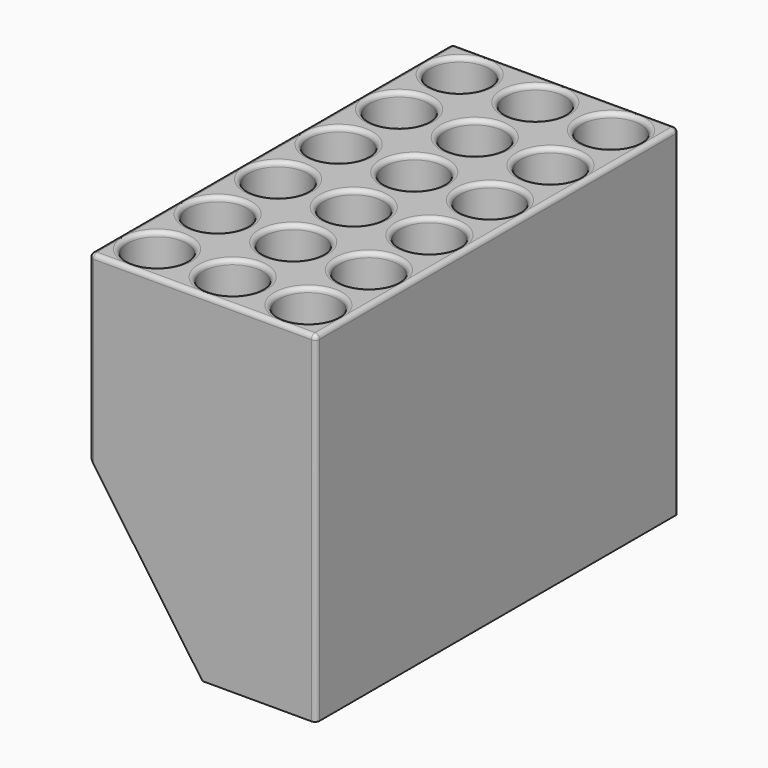
from build123d import *

# Parameters (mm, degrees)
F1_DEPTH     = 100
F2_R         = 6.5
F3_DEPTH     = 60
F4_R         = 6.5
F5_DEPTH     = 60
F6_R         = 6.5
F7_DEPTH     = 37
F8_T1_DEPTH  = 98
F8_T3_DEPTH  = 48
F8_T5_DEPTH  = 76.5
F8_T7_DEPTH  = 40.7962998314
F8_S11_W     = 1
F8_S11_H     = 1
F8_T12_DEPTH = 1
F8_S17_W     = 1
F8_S17_H     = 1
F8_T18_DEPTH = 1
F8_S23_W     = 1
F8_S23_H     = 1
F8_T24_DEPTH = 1
F8_S29_W     = 1
F8_S29_H     = 1
F8_T30_DEPTH = 1


# Not quite as in the source:
# - a fillet or chamfer that OpenCascade refuses, or shapes differently, is made with other operations: its cross-section is extruded or revolved along the edge and cut away or added


with BuildPart() as f1:
    # F0 (on Front) → F1 (new body)
    with BuildSketch(Plane.XZ):
        Polygon((0, 35.7037001686), (25, 0), (50, 0), (50, 75), (0, 75), align=None)
    extrude(amount=F1_DEPTH)

    # F2 (on face) → F3 (cut)
    with BuildSketch(Plane.XY.offset(75)):
        with Locations((41.667, -8.333)):
            Circle(F2_R)
        with Locations((41.667, -25)):
            Circle(F2_R)
        with Locations((41.667, -41.667)):
            Circle(F2_R)
        with Locations((41.667, -58.334)):
            Circle(F2_R)
        with Locations((41.667, -75.001)):
            Circle(F2_R)
        with Locations((41.667, -91.668)):
            Circle(F2_R)
    extrude(amount=-F3_DEPTH, mode=Mode.SUBTRACT)

    # F4 (on face) → F5 (cut)
    with BuildSketch(Plane.XY.offset(75)):
        with Locations((25, -8.333)):
            Circle(F4_R)
        with Locations((25, -25)):
            Circle(F4_R)
        with Locations((25, -41.667)):
            Circle(F4_R)
        with Locations((25, -58.334)):
            Circle(F4_R)
        with Locations((25, -75.001)):
            Circle(F4_R)
        with Locations((25, -91.668)):
            Circle(F4_R)
    extrude(amount=-F5_DEPTH, mode=Mode.SUBTRACT)

    # F6 (on face) → F7 (cut)
    with BuildSketch(Plane.XY.offset(75)):
        with Locations((8.333, -8.333)):
            Circle(F6_R)
        with Locations((8.333, -25)):
            Circle(F6_R)
        with Locations((8.333, -41.667)):
            Circle(F6_R)
        with Locations((8.333, -58.334)):
            Circle(F6_R)
        with Locations((8.333, -75.001)):
            Circle(F6_R)
        with Locations((8.333, -91.668)):
            Circle(F6_R)
    extrude(amount=-F7_DEPTH, mode=Mode.SUBTRACT)

    # F8: fillet of radius 1 on 26 edges, made by hand

    # F8_s2 → F8_t1 (cut)
    with BuildSketch(Plane.XZ.offset(1)):
        with BuildLine():
            ThreePointArc((49, 75), (49.7071067812, 74.7071067812), (50, 74))
            Line((50, 74), (50, 75))
            Line((50, 75), (49, 75))
        make_face()
        with BuildLine():
            ThreePointArc((0, 74), (0.2928932188, 74.7071067812), (1, 75))
            Line((1, 75), (0, 75))
            Line((0, 75), (0, 74))
        make_face()
    extrude(amount=F8_T1_DEPTH, mode=Mode.SUBTRACT)

    # F8_s4 → F8_t3 (cut)
    with BuildSketch(Plane.YZ.offset(1)):
        with BuildLine():
            ThreePointArc((0, 74), (-0.2928932188, 74.7071067812), (-1, 75))
            Line((-1, 75), (0, 75))
            Line((0, 75), (0, 74))
        make_face()
        with BuildLine():
            ThreePointArc((-100, 74), (-99.7071067812, 74.7071067812), (-99, 75))
            Line((-99, 75), (-100, 75))
            Line((-100, 75), (-100, 74))
        make_face()
    extrude(amount=F8_T3_DEPTH, mode=Mode.SUBTRACT)

    # F8_s6 → F8_t5 (cut)
    with BuildSketch(Plane.XY.offset(-2.5)):
        with BuildLine():
            ThreePointArc((49, -100), (49.7071067812, -99.7071067812), (50, -99))
            Line((50, -99), (50, -100))
            Line((50, -100), (49, -100))
        make_face()
        with BuildLine():
            ThreePointArc((49, 0), (49.7071067812, -0.2928932188), (50, -1))
            Line((50, -1), (50, 0))
            Line((50, 0), (49, 0))
        make_face()
    extrude(amount=F8_T5_DEPTH, mode=Mode.SUBTRACT)

    # F8_s8 → F8_t7 (cut)
    with BuildSketch(Plane.XY.offset(33.2037001686)):
        with BuildLine():
            ThreePointArc((0, -99), (0.2928932188, -99.7071067812), (1, -100))
            Line((1, -100), (0, -100))
            Line((0, -100), (0, -99))
        make_face()
        with BuildLine():
            ThreePointArc((0, -1), (0.2928932188, -0.2928932188), (1, 0))
            Line((1, 0), (0, 0))
            Line((0, 0), (0, -1))
        make_face()
    extrude(amount=F8_T7_DEPTH, mode=Mode.SUBTRACT)


with BuildPart() as f8_tool10:
    # F8_s11 → F8_t12 (new body)
    with BuildSketch(Plane.XZ.offset(1)):
        with Locations((49.5, 74.5)):
            Rectangle(F8_S11_W, F8_S11_H)
    extrude(amount=-F8_T12_DEPTH)

    # F8_s13 → F8_t14 (revolve, cut)
    with BuildSketch(Plane(origin=(49, -1, 74), x_dir=(-0.7071067812, 0, -0.7071067812), z_dir=(0.7071067812, 0, -0.7071067812))):
        with BuildLine():
            ThreePointArc((0, -1), (1, 0), (0, 1))
            Line((0, 1), (0, -1))
        make_face()
    revolve(axis=Axis((49, -1, 74), (0, 1, 0)), mode=Mode.SUBTRACT)


with BuildPart() as f1_1:
    add(f1.part)

    # F8_t9: cut F8_tool10
    add(f8_tool10.part, mode=Mode.SUBTRACT)


with BuildPart() as f8_tool16:
    # F8_s17 → F8_t18 (new body)
    with BuildSketch(Plane.XZ.offset(99)):
        with Locations((49.5, 74.5)):
            Rectangle(F8_S17_W, F8_S17_H)
    extrude(amount=F8_T18_DEPTH)

    # F8_s19 → F8_t20 (revolve, cut)
    with BuildSketch(Plane(origin=(49, -99, 74), x_dir=(-0.7071067812, 0, -0.7071067812), z_dir=(-0.7071067812, 0, 0.7071067812))):
        with BuildLine():
            ThreePointArc((0, -1), (1, 0), (0, 1))
            Line((0, 1), (0, -1))
        make_face()
    revolve(axis=Axis((49, -99, 74), (0, -1, 0)), mode=Mode.SUBTRACT)


with BuildPart() as f1_2:
    add(f1_1.part)

    # F8_t15: cut F8_tool16
    add(f8_tool16.part, mode=Mode.SUBTRACT)


with BuildPart() as f8_tool22:
    # F8_s23 → F8_t24 (new body)
    with BuildSketch(Plane.YZ.offset(1)):
        with Locations((-0.5, 74.5)):
            Rectangle(F8_S23_W, F8_S23_H)
    extrude(amount=-F8_T24_DEPTH)

    # F8_s25 → F8_t26 (revolve, cut)
    with BuildSketch(Plane(origin=(1, -1, 74), x_dir=(0, -0.7071067812, -0.7071067812), z_dir=(0, 0.7071067812, -0.7071067812))):
        with BuildLine():
            ThreePointArc((0, -1), (1, 0), (0, 1))
            Line((0, 1), (0, -1))
        make_face()
    revolve(axis=Axis((1, -1, 74), (-1, 0, 0)), mode=Mode.SUBTRACT)


with BuildPart() as f1_3:
    add(f1_2.part)

    # F8_t21: cut F8_tool22
    add(f8_tool22.part, mode=Mode.SUBTRACT)


with BuildPart() as f8_tool28:
    # F8_s29 → F8_t30 (new body)
    with BuildSketch(Plane.YZ.offset(1)):
        with Locations((-99.5, 74.5)):
            Rectangle(F8_S29_W, F8_S29_H)
    extrude(amount=-F8_T30_DEPTH)

    # F8_s31 → F8_t32 (revolve, cut)
    with BuildSketch(Plane(origin=(1, -99, 74), x_dir=(0, 0.7071067812, -0.7071067812), z_dir=(0, 0.7071067812, 0.7071067812))):
        with BuildLine():
            ThreePointArc((0, -1), (1, 0), (0, 1))
            Line((0, 1), (0, -1))
        make_face()
    revolve(axis=Axis((1, -99, 74), (-1, 0, 0)), mode=Mode.SUBTRACT)


with BuildPart() as f1_4:
    add(f1_3.part)

    # F8_t27: cut F8_tool28
    add(f8_tool28.part, mode=Mode.SUBTRACT)

    # F8_s33 → F8_t34 (revolve, cut)
    with BuildSketch(Plane.XZ.offset(91.668)):
        with BuildLine():
            ThreePointArc((49.167, 75), (48.4598932188, 74.7071067812), (48.167, 74))
            Line((48.167, 74), (48.167, 75))
            Line((48.167, 75), (49.167, 75))
        make_face()
    revolve(axis=Axis((41.667, -91.668, 75), (0, 0, 1)), mode=Mode.SUBTRACT)

    # F8_s35 → F8_t36 (revolve, cut)
    with BuildSketch(Plane.XZ.offset(75.001)):
        with BuildLine():
            ThreePointArc((49.167, 75), (48.4598932188, 74.7071067812), (48.167, 74))
            Line((48.167, 74), (48.167, 75))
            Line((48.167, 75), (49.167, 75))
        make_face()
    revolve(axis=Axis((41.667, -75.001, 75), (0, 0, 1)), mode=Mode.SUBTRACT)

    # F8_s37 → F8_t38 (revolve, cut)
    with BuildSketch(Plane.XZ.offset(58.334)):
        with BuildLine():
            ThreePointArc((49.167, 75), (48.4598932188, 74.7071067812), (48.167, 74))
            Line((48.167, 74), (48.167, 75))
            Line((48.167, 75), (49.167, 75))
        make_face()
    revolve(axis=Axis((41.667, -58.334, 75), (0, 0, 1)), mode=Mode.SUBTRACT)

    # F8_s39 → F8_t40 (revolve, cut)
    with BuildSketch(Plane.XZ.offset(91.668)):
        with BuildLine():
            ThreePointArc((32.5, 75), (31.7928932188, 74.7071067812), (31.5, 74))
            Line((31.5, 74), (31.5, 75))
            Line((31.5, 75), (32.5, 75))
        make_face()
    revolve(axis=Axis((25, -91.668, 75), (0, 0, 1)), mode=Mode.SUBTRACT)

    # F8_s41 → F8_t42 (revolve, cut)
    with BuildSketch(Plane.XZ.offset(75.001)):
        with BuildLine():
            ThreePointArc((32.5, 75), (31.7928932188, 74.7071067812), (31.5, 74))
            Line((31.5, 74), (31.5, 75))
            Line((31.5, 75), (32.5, 75))
        make_face()
    revolve(axis=Axis((25, -75.001, 75), (0, 0, 1)), mode=Mode.SUBTRACT)

    # F8_s43 → F8_t44 (revolve, cut)
    with BuildSketch(Plane.XZ.offset(91.668)):
        with BuildLine():
            ThreePointArc((15.833, 75), (15.1258932188, 74.7071067812), (14.833, 74))
            Line((14.833, 74), (14.833, 75))
            Line((14.833, 75), (15.833, 75))
        make_face()
    revolve(axis=Axis((8.333, -91.668, 75), (0, 0, 1)), mode=Mode.SUBTRACT)

    # F8_s45 → F8_t46 (revolve, cut)
    with BuildSketch(Plane.XZ.offset(75.001)):
        with BuildLine():
            ThreePointArc((15.833, 75), (15.1258932188, 74.7071067812), (14.833, 74))
            Line((14.833, 74), (14.833, 75))
            Line((14.833, 75), (15.833, 75))
        make_face()
    revolve(axis=Axis((8.333, -75.001, 75), (0, 0, 1)), mode=Mode.SUBTRACT)

    # F8_s47 → F8_t48 (revolve, cut)
    with BuildSketch(Plane.XZ.offset(58.334)):
        with BuildLine():
            ThreePointArc((32.5, 75), (31.7928932188, 74.7071067812), (31.5, 74))
            Line((31.5, 74), (31.5, 75))
            Line((31.5, 75), (32.5, 75))
        make_face()
    revolve(axis=Axis((25, -58.334, 75), (0, 0, 1)), mode=Mode.SUBTRACT)

    # F8_s49 → F8_t50 (revolve, cut)
    with BuildSketch(Plane.XZ.offset(58.334)):
        with BuildLine():
            ThreePointArc((15.833, 75), (15.1258932188, 74.7071067812), (14.833, 74))
            Line((14.833, 74), (14.833, 75))
            Line((14.833, 75), (15.833, 75))
        make_face()
    revolve(axis=Axis((8.333, -58.334, 75), (0, 0, 1)), mode=Mode.SUBTRACT)

    # F8_s51 → F8_t52 (revolve, cut)
    with BuildSketch(Plane.XZ.offset(41.667)):
        with BuildLine():
            ThreePointArc((49.167, 75), (48.4598932188, 74.7071067812), (48.167, 74))
            Line((48.167, 74), (48.167, 75))
            Line((48.167, 75), (49.167, 75))
        make_face()
    revolve(axis=Axis((41.667, -41.667, 75), (0, 0, 1)), mode=Mode.SUBTRACT)

    # F8_s53 → F8_t54 (revolve, cut)
    with BuildSketch(Plane.XZ.offset(25)):
        with BuildLine():
            ThreePointArc((49.167, 75), (48.4598932188, 74.7071067812), (48.167, 74))
            Line((48.167, 74), (48.167, 75))
            Line((48.167, 75), (49.167, 75))
        make_face()
    revolve(axis=Axis((41.667, -25, 75), (0, 0, 1)), mode=Mode.SUBTRACT)

    # F8_s55 → F8_t56 (revolve, cut)
    with BuildSketch(Plane.XZ.offset(8.333)):
        with BuildLine():
            ThreePointArc((49.167, 75), (48.4598932188, 74.7071067812), (48.167, 74))
            Line((48.167, 74), (48.167, 75))
            Line((48.167, 75), (49.167, 75))
        make_face()
    revolve(axis=Axis((41.667, -8.333, 75), (0, 0, 1)), mode=Mode.SUBTRACT)

    # F8_s57 → F8_t58 (revolve, cut)
    with BuildSketch(Plane.XZ.offset(41.667)):
        with BuildLine():
            ThreePointArc((32.5, 75), (31.7928932188, 74.7071067812), (31.5, 74))
            Line((31.5, 74), (31.5, 75))
            Line((31.5, 75), (32.5, 75))
        make_face()
    revolve(axis=Axis((25, -41.667, 75), (0, 0, 1)), mode=Mode.SUBTRACT)

    # F8_s59 → F8_t60 (revolve, cut)
    with BuildSketch(Plane.XZ.offset(41.667)):
        with BuildLine():
            ThreePointArc((15.833, 75), (15.1258932188, 74.7071067812), (14.833, 74))
            Line((14.833, 74), (14.833, 75))
            Line((14.833, 75), (15.833, 75))
        make_face()
    revolve(axis=Axis((8.333, -41.667, 75), (0, 0, 1)), mode=Mode.SUBTRACT)

    # F8_s61 → F8_t62 (revolve, cut)
    with BuildSketch(Plane.XZ.offset(25)):
        with BuildLine():
            ThreePointArc((32.5, 75), (31.7928932188, 74.7071067812), (31.5, 74))
            Line((31.5, 74), (31.5, 75))
            Line((31.5, 75), (32.5, 75))
        make_face()
    revolve(axis=Axis((25, -25, 75), (0, 0, 1)), mode=Mode.SUBTRACT)

    # F8_s63 → F8_t64 (revolve, cut)
    with BuildSketch(Plane.XZ.offset(8.333)):
        with BuildLine():
            ThreePointArc((32.5, 75), (31.7928932188, 74.7071067812), (31.5, 74))
            Line((31.5, 74), (31.5, 75))
            Line((31.5, 75), (32.5, 75))
        make_face()
    revolve(axis=Axis((25, -8.333, 75), (0, 0, 1)), mode=Mode.SUBTRACT)

    # F8_s65 → F8_t66 (revolve, cut)
    with BuildSketch(Plane.XZ.offset(25)):
        with BuildLine():
            ThreePointArc((15.833, 75), (15.1258932188, 74.7071067812), (14.833, 74))
            Line((14.833, 74), (14.833, 75))
            Line((14.833, 75), (15.833, 75))
        make_face()
    revolve(axis=Axis((8.333, -25, 75), (0, 0, 1)), mode=Mode.SUBTRACT)

    # F8_s67 → F8_t68 (revolve, cut)
    with BuildSketch(Plane.XZ.offset(8.333)):
        with BuildLine():
            ThreePointArc((15.833, 75), (15.1258932188, 74.7071067812), (14.833, 74))
            Line((14.833, 74), (14.833, 75))
            Line((14.833, 75), (15.833, 75))
        make_face()
    revolve(axis=Axis((8.333, -8.333, 75), (0, 0, 1)), mode=Mode.SUBTRACT)


solid = f1_4.part
